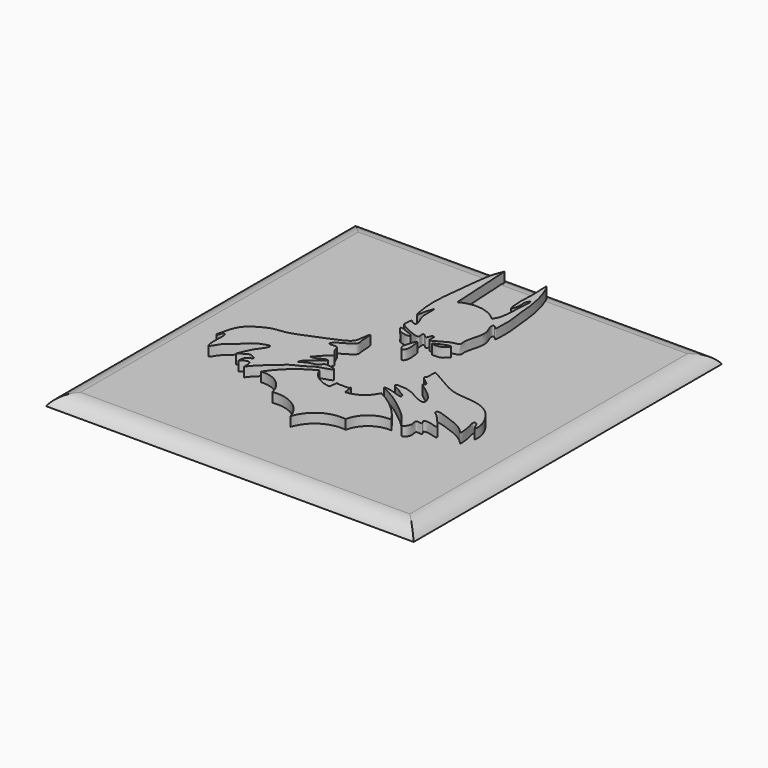
from build123d import *

# Parameters (mm, degrees)
F1_DEPTH    = 8.636
F0_W        = 157.6474606991
F0_H        = 165.2397401631
F2_DEPTH    = 4.572
F3_T1_DEPTH = 199.1265994465
F3_T3_DEPTH = 206.7188789105


# Not quite as in the source:
# - a fillet or chamfer that OpenCascade refuses, or shapes differently, is made with other operations: its cross-section is extruded or revolved along the edge and cut away or added


with BuildPart() as f1:
    # F0 (on Top) → F1 (new body)
    with BuildSketch(Plane.XY):
        with BuildLine():
            Line((-8.0563426018, 32.0382602513), (-9.5873847604, 59.3079030514))
            add(Edge.make_bspline(
                [(-9.5873847604, 59.3079030514), (-10.2069740501, 57.8510791752), (-11.6288952228, 54.5077536066), (-12.571011767, 45.9160526153), (-13.8278968188, 35.8790758133), (-14.8130812466, 24.4032074281), (-12.6930088149, 14.2813385529), (-12.4467480347, 19.5686321405), (-11.3588516792, 22.1258498776), (-10.9689455739, 23.9673491113), (-10.7703404995, 22.210055132), (-10.8849088261, 20.4345795664), (-10.8702437558, 16.7478927392), (-9.9164388242, 14.4470348521), (-8.9093176999, 12.4710831019), (-8.8130882414, 10.5507668204), (-10.0726759825, 11.0809174378), (-11.1105414789, 11.4684363429), (-11.5467394355, 12.4794641642), (-12.0326045569, 11.1352392958), (-12.0718164854, 9.0656207612), (-12.1678725214, 7.8042704483), (-1.7397194602, 2.850652627), (-2.7152347011, 5.6312047686), (-2.6333232506, 7.0837245523), (-1.5405587064, 6.595512113), (-0.3523573577, 5.1847846555), (0.0176657446, 6.1495776898), (0.3440615571, 6.8678292671), (0.6920890595, 7.6887216528), (1.7445455533, 7.8221392033), (1.6925707752, 6.6794200294), (1.5694466399, 5.9493515122), (1.7384837371, 5.3483126386), (1.7238072902, 4.2958486754), (4.2518249694, 5.5379971352), (7.5388645263, 7.6288405278), (9.5491214189, 8.2193902514), (12.1832042354, 8.6803960253), (11.2527745874, 11.5048248524), (12.9626901314, 16.4433777124), (13.6012979663, 21.5049566899), (11.6736068309, 24.314855315), (11.7201059386, 26.9225111344), (13.2570231691, 25.7198167097), (14.0571000334, 24.3610756973), (14.1651481676, 28.6480973338), (14.2838550528, 32.7466596802), (13.191654245, 38.6947421466), (13.0597426804, 43.5898107344), (11.6516605619, 52.5903286162), (7.7032874495, 61.6806237813), (8.3342558909, 55.6029864465), (8.3560371943, 48.142569085), (7.9148713681, 45.9656915319), (8.3982670386, 41.7710296595), (8.7042650126, 38.596342426), (10.3088253456, 43.154016532), (9.3465585879, 45.7452585782), (11.2795851261, 48.6649542065), (10.9361180212, 44.1687097023), (10.5666606894, 40.3809380114), (10.4802282511, 32.4778899259), (8.6848033832, 30.3255504932), (8.5917155195, 29.9147238101), (8.5641695186, 29.7931544483)],
                knots=[0, 0, 0, 0, 0.0215680204, 0.0494973451, 0.0803067556, 0.1149771587, 0.1397760921, 0.1556042663, 0.173574449, 0.1833185564, 0.1930074754, 0.2067732445, 0.2250113268, 0.2403192089, 0.2549776383, 0.2662207325, 0.2755793133, 0.2862530722, 0.2940626367, 0.3034624078, 0.3174077042, 0.3281447576, 0.3578417858, 0.368882565, 0.3793332655, 0.3883559951, 0.400307943, 0.4079673083, 0.4169542407, 0.425807678, 0.4339422803, 0.4431398948, 0.4516444118, 0.4593494611, 0.4669484468, 0.4812481254, 0.5008700638, 0.5152502277, 0.5289135867, 0.5433599989, 0.5656053014, 0.5871321546, 0.6049528358, 0.6172889038, 0.6286238669, 0.6374714134, 0.6542574113, 0.6752363731, 0.698287396, 0.7195672617, 0.7501912632, 0.7750519975, 0.7925526419, 0.8197608492, 0.8345022352, 0.8547565152, 0.8673256205, 0.8844942075, 0.9019948421, 0.9149074029, 0.9308938897, 0.9517413657, 0.9785266178, 0.9936457258, 1, 1, 1, 1], degree=3))
            ThreePointArc((8.5641695186, 29.7931544483), (0.6273246637, 33.6800694814), (-8.0563426018, 32.0382602513))
        make_face()
    extrude(amount=F1_DEPTH)


with BuildPart() as f1b:
    # F0 (on Top) → F1, piece 2 (new body)
    with BuildSketch(Plane.XY):
        with BuildLine():
            add(Edge.make_bspline(
                [(-11.3129224628, 5.8338870294), (-11.212077991, 6.0836919569), (-9.5446702313, 5.498751424), (-7.6526266007, 4.7544780652), (-4.8522655809, 3.7151044125), (-5.6744214857, 2.3720213293), (-8.5846141026, 3.1775841412), (-9.7788566178, 3.3609961858), (-11.4458218222, 5.5046779591), (-11.3129224628, 5.8338870294)],
                knots=[0, 0, 0, 0, 0.1234585709, 0.2884281256, 0.4484905967, 0.5401562643, 0.7088422597, 0.83729832, 1, 1, 1, 1], degree=3))
        make_face()
    extrude(amount=F1_DEPTH)


with BuildPart() as f1c:
    # F0 (on Top) → F1, piece 3 (new body)
    with BuildSketch(Plane.XY):
        with BuildLine():
            add(Edge.make_bspline(
                [(4.2034736834, 3.2082463149), (4.1171338962, 3.3867294322), (5.3945718393, 4.2279527832), (7.871360839, 5.2078627509), (9.5517951768, 5.8839128476), (10.8777071041, 5.6073678199), (9.2708457074, 4.4751151628), (8.2710626919, 3.2190418207), (6.3604336283, 3.0183269191), (4.3102453409, 2.9875260782), (4.2034736834, 3.2082463149)],
                knots=[0, 0, 0, 0, 0.1086692497, 0.274727001, 0.406939114, 0.4888761294, 0.6034499567, 0.727631672, 0.8656147266, 1, 1, 1, 1], degree=3))
        make_face()
    extrude(amount=F1_DEPTH)


with BuildPart() as f1d:
    # F0 (on Top) → F1, piece 4 (new body)
    with BuildSketch(Plane.XY):
        with BuildLine():
            add(Edge.make_bspline(
                [(-0.4922925145, 1.1984186713), (-0.7219822659, 1.2413124065), (-1.5725812282, -0.1617702452), (-1.8935343811, -2.3371597334), (-2.5761843842, -3.8672516478), (-2.3162609098, -5.1141898438), (-1.0121639923, -6.7835477453), (0.4038948302, -4.6520691166), (-0.0283463576, -1.1777215689), (-0.0962722826, 0.1357641207), (-0.3086551187, 1.1641250479), (-0.4922925145, 1.1984186713)],
                knots=[0, 0, 0, 0, 0.102513173, 0.2351976422, 0.3413296648, 0.4367849301, 0.5411400619, 0.6544107074, 0.8137842706, 0.918040522, 1, 1, 1, 1], degree=3))
        make_face()
    extrude(amount=F1_DEPTH)


with BuildPart() as f1e:
    # F0 (on Top) → F1, piece 5 (new body)
    with BuildSketch(Plane.XY):
        with BuildLine():
            add(Edge.make_bspline(
                [(-56.5317720175, -36.4757142961), (-56.3085275842, -35.3899332292), (-55.7960366931, -32.8885452847), (-54.0426175772, -26.7831440592), (-48.5321006344, -23.2926451301), (-44.5299851578, -21.2785733802), (-37.744733397, -21.0053075427), (-30.8060554473, -17.4194604059), (-18.5940164844, -13.2184714608), (-16.8743985097, -10.1721897893), (-16.9012842846, -7.8020298205), (-15.8976571712, -3.1934213643), (-15.8006185861, -7.4747740916), (-15.7020221735, -9.8808797844), (-15.036609521, -11.83844459), (-16.4503720124, -13.4391939901), (-20.0262562132, -15.3997435363), (-21.8881261976, -16.2977734279), (-23.3955349466, -18.4890981482), (-21.0565555139, -18.3918166801), (-19.0412600912, -18.140499788), (-18.8028673653, -19.8230302625), (-17.818011388, -21.6935992037), (-17.1193392555, -22.3536708663), (-15.7073878024, -24.0554988779), (-18.7233056749, -25.7252328416), (-20.3645373071, -28.354481793), (-22.8099407509, -29.9214724173), (-18.7229926684, -29.1680810509), (-17.5001874468, -27.941324871), (-14.3629528526, -27.486134602), (-18.6008603941, -30.3633212973), (-20.0842758034, -31.8567752366), (-21.9914900575, -32.9897828812), (-23.3175952088, -35.9553450316), (-19.9363871131, -32.9237966924), (-15.3834104243, -32.8316576362), (-15.2787570435, -30.6204718377), (-12.5601866802, -30.5905559397), (-8.5162795966, -31.8659123733), (-12.8665495258, -33.1359132687), (-16.3544489489, -34.1340040074), (-19.6077369159, -36.8480297152), (-23.9258639487, -38.2572226049), (-26.4016508932, -41.3086310679), (-29.889560769, -43.7575731288), (-33.2428135147, -47.1877803235), (-34.2014949385, -48.5179926444), (-34.5914438367, -49.0590669215)],
                knots=[0, 0, 0, 0, 0.0235054063, 0.0541714038, 0.0851440949, 0.111308795, 0.14222986, 0.1783242724, 0.2222777227, 0.2433825477, 0.2637111406, 0.2847053536, 0.3040919602, 0.3252304726, 0.3416503728, 0.3587446101, 0.3837110785, 0.4027046969, 0.4189237643, 0.434797145, 0.4516974638, 0.4663698249, 0.4842223365, 0.4970387457, 0.5124994639, 0.5331958128, 0.5567519831, 0.5718107872, 0.5922051865, 0.6111406286, 0.6263819983, 0.6496852012, 0.6694935076, 0.6882990399, 0.7047724597, 0.7262713232, 0.7524047523, 0.7671438816, 0.786982741, 0.807561723, 0.8283115693, 0.8533238079, 0.8784768485, 0.9045011258, 0.9285856605, 0.9544829455, 0.9815143267, 1, 1, 1, 1], degree=3))
            add(Edge.make_bspline(
                [(-34.5914438367, -49.0590669215), (-34.5617406662, -48.4645916409), (-34.5015091034, -47.2550371222), (-34.9231333712, -45.2879063315), (-36.6352958616, -45.0185438688), (-38.1275834761, -46.4156266116), (-39.0504091016, -47.1771096694), (-38.6387314573, -45.3877670548), (-38.4250127074, -43.1979119569), (-34.7845880016, -42.5577217331), (-37.7439039605, -40.9493748194), (-38.7560351456, -40.7890446139), (-40.8150603497, -42.1673004931), (-42.0745475807, -42.6956108287), (-42.8998646706, -43.8533010921), (-41.7082013729, -41.02927019), (-40.0292794785, -37.0379365322), (-37.3109398728, -33.9222730739), (-36.7235339468, -31.6524819302), (-38.8601120182, -31.9042472556), (-43.7324241455, -34.0352374035), (-46.2025642266, -37.594436589), (-49.9657372312, -40.1469617994), (-51.5753222919, -42.1336066798), (-53.3116998576, -45.5754431201), (-54.11435487, -42.6530847524), (-54.0795511785, -39.8375115199), (-53.9142722396, -36.9687224915), (-53.9337726693, -35.9541859846), (-54.3444092876, -34.0062490401), (-55.8776571006, -35.4763912856), (-55.773981613, -37.14106453), (-56.3128012293, -36.6679736125), (-56.5317720175, -36.4757142961)],
                knots=[0, 0, 0, 0, 0.0306089862, 0.0605779455, 0.0867220518, 0.119466043, 0.1379441871, 0.1633760962, 0.1971675416, 0.2306435809, 0.2632017867, 0.2874606202, 0.3216074169, 0.3496849568, 0.3678851507, 0.3995177636, 0.4492656593, 0.4956544404, 0.524008621, 0.55106341, 0.6027475455, 0.6504689503, 0.69697749, 0.735409776, 0.7717076052, 0.801572517, 0.8420773346, 0.8791897934, 0.9034034657, 0.9292672177, 0.9565885872, 0.981875991, 1, 1, 1, 1], degree=3))
        make_face()
    extrude(amount=F1_DEPTH)


with BuildPart() as f1f:
    # F0 (on Top) → F1, piece 6 (new body)
    with BuildSketch(Plane.XY):
        with BuildLine():
            add(Edge.make_bspline(
                [(11.3561199978, -31.5462760627), (11.2708232902, -31.8494182358), (17.1916397479, -34.2819237216), (22.8631387434, -38.8349813838), (29.8063616714, -44.1603330844), (33.1387713155, -50.1267706744), (34.5396741163, -48.8557368561), (35.4714882721, -47.213305576), (35.3042623997, -45.7627282077), (34.7935519176, -44.0431695576), (36.1375577984, -43.7628594372), (37.8716341978, -44.30387013), (37.4190158392, -43.159612785), (36.3824914624, -42.1406612695), (38.6318730978, -41.8072170173), (40.1553549966, -42.164726162), (44.0894732797, -43.5380661341), (41.4220220506, -40.4700964927), (39.3518408463, -38.0199885713), (37.3515430903, -35.8618404922), (35.9013185364, -35.1833512057), (36.3078265927, -33.5728204552), (39.4561495274, -34.6972965204), (44.3510012501, -36.2798979776), (50.0337333297, -38.8662677252), (52.1223899971, -42.0264216155), (51.989348781, -39.5219509981), (51.6582572588, -37.3685552937), (51.3032706529, -35.4106328984), (50.3378532171, -32.622045103), (51.7855547632, -32.2974748095), (52.6049629965, -33.6698853924), (53.9423638795, -37.048777693), (54.2409254928, -33.1267342607), (52.3854787877, -28.1337374698), (47.9530116507, -22.6083548802), (41.331769958, -20.5112354176), (35.05419088, -20.3961087662), (29.6940561643, -19.098259547), (24.1383301141, -15.832340626), (18.6607055154, -12.5331934369), (18.1259123911, -12.4097767417), (17.9909168325, -13.1479184713), (17.9535379241, -14.4114186042), (18.0676703856, -15.7004041283), (17.9260726891, -17.0669513695), (17.0850166317, -17.2757653009), (18.095102178, -18.4661333892), (19.9339732524, -19.6693085298), (21.1709176908, -20.8449222954), (20.8552869509, -21.7922559491), (19.5396603619, -21.5424004948), (21.1406348542, -22.760811599), (22.889906786, -23.8290796941), (24.9307608472, -25.6037416108), (25.3058857425, -25.7541587946), (27.2535142167, -27.7773825531), (27.5456715584, -28.0711397096), (28.3645450501, -29.6113323522), (28.9491463629, -31.2233535764), (27.7615827313, -31.9665108042), (25.6796017707, -31.1125851813), (23.7189459148, -30.3195990814), (20.868861509, -28.4078463352), (17.3597853751, -27.4504491891), (16.3649111705, -27.5741175461), (15.1791383287, -27.4827337621), (13.293302009, -27.2752369899), (13.2771080651, -28.8255516731), (16.4679377367, -29.5237431729), (17.6955882572, -31.2418041093), (19.902172027, -31.7891686271), (20.3497248586, -34.0562482813), (14.6119485045, -31.4979431235), (13.034312592, -31.4892860499), (11.3983533668, -31.3961798209), (11.3561199978, -31.5462760627)],
                knots=[0, 0, 0, 0, 0.0207712469, 0.0468010185, 0.0740281994, 0.0953806066, 0.1048831637, 0.1171105979, 0.1281810161, 0.1390164492, 0.1484333243, 0.1590379808, 0.1670070375, 0.1760829796, 0.1871520185, 0.2002205864, 0.2147618528, 0.2286747001, 0.2461395079, 0.2614180487, 0.2719585888, 0.2806602226, 0.2953583218, 0.3165908605, 0.3397066295, 0.3534940351, 0.3643098423, 0.3781409522, 0.3914439389, 0.405697964, 0.4137994303, 0.4254296768, 0.4393008252, 0.4524650877, 0.4739550989, 0.4974999134, 0.5208073503, 0.543208937, 0.5638870529, 0.5877483837, 0.6097735957, 0.6146449264, 0.6215906595, 0.6318524469, 0.6424545507, 0.6524798852, 0.6589274487, 0.6685474208, 0.6826281714, 0.6938838396, 0.701344386, 0.7089221438, 0.7188362561, 0.7331597297, 0.7472245684, 0.7538431679, 0.7683767168, 0.7749596765, 0.7865937658, 0.7978733074, 0.806796258, 0.8198580259, 0.8330984023, 0.8500047315, 0.8668764886, 0.8755687455, 0.8855328188, 0.8969508767, 0.9051905148, 0.9206295997, 0.9339190842, 0.9469970149, 0.9559339563, 0.9762144194, 0.9897154327, 1, 1, 1, 1], degree=3))
        make_face()
    extrude(amount=F1_DEPTH)


with BuildPart() as f1g:
    # F0 (on Top) → F1, piece 7 (new body)
    with BuildSketch(Plane.XY):
        with BuildLine():
            ThreePointArc((-3.3188456437, -42.3583795704), (-9.3072729106, -40.3191361107), (-13.2902822224, -35.4043205657))
            ThreePointArc((-13.2902822224, -35.4043205657), (-21.481283067, -40.8505875442), (-27.9277319787, -48.2800973036))
            ThreePointArc((-27.9277319787, -48.2800973036), (-20.0606479541, -50.5503244222), (-15.7425979851, -57.5072911956))
            ThreePointArc((-15.7425979851, -57.5072911956), (-6.0369640986, -59.5197584467), (0, -67.3813370444))
            ThreePointArc((0, -67.3813370444), (6.0369640986, -59.5197584467), (15.7425979851, -57.5072911956))
            ThreePointArc((15.7425979851, -57.5072911956), (20.0606479541, -50.5503244222), (27.9277319787, -48.2800973036))
            ThreePointArc((27.9277319787, -48.2800973036), (21.481283067, -40.8505875442), (13.2902822224, -35.4043205657))
            ThreePointArc((13.2902822224, -35.4043205657), (9.3072729106, -40.3191361107), (3.3188456437, -42.3583795704))
            Line((3.3188456437, -42.3583795704), (2.8344087768, -38.5856293142))
            Line((2.8344087768, -38.5856293142), (2.3823640459, -39.2272426674))
            Line((2.3823640459, -39.2272426674), (0, -39.2272426674))
            Line((0, -39.2272426674), (-2.3823640459, -39.2272426674))
            Line((-2.3823640459, -39.2272426674), (-2.8344087768, -38.5856293142))
            Line((-2.8344087768, -38.5856293142), (-3.3188456437, -42.3583795704))
        make_face()
    extrude(amount=F1_DEPTH)


with BuildPart() as f2:
    # F0 (on Top) → F2 (new body)
    with BuildSketch(Plane.XY):
        with Locations((0, -17.3164587468)):
            Rectangle(F0_W, F0_H)
        with BuildLine():
            add(Edge.make_bspline(
                [(-34.5914438367, -49.0590669215), (-34.5617406662, -48.4645916409), (-34.5015091034, -47.2550371222), (-34.9231333712, -45.2879063315), (-36.6352958616, -45.0185438688), (-38.1275834761, -46.4156266116), (-39.0504091016, -47.1771096694), (-38.6387314573, -45.3877670548), (-38.4250127074, -43.1979119569), (-34.7845880016, -42.5577217331), (-37.7439039605, -40.9493748194), (-38.7560351456, -40.7890446139), (-40.8150603497, -42.1673004931), (-42.0745475807, -42.6956108287), (-42.8998646706, -43.8533010921), (-41.7082013729, -41.02927019), (-40.0292794785, -37.0379365322), (-37.3109398728, -33.9222730739), (-36.7235339468, -31.6524819302), (-38.8601120182, -31.9042472556), (-43.7324241455, -34.0352374035), (-46.2025642266, -37.594436589), (-49.9657372312, -40.1469617994), (-51.5753222919, -42.1336066798), (-53.3116998576, -45.5754431201), (-54.11435487, -42.6530847524), (-54.0795511785, -39.8375115199), (-53.9142722396, -36.9687224915), (-53.9337726693, -35.9541859846), (-54.3444092876, -34.0062490401), (-55.8776571006, -35.4763912856), (-55.773981613, -37.14106453), (-56.3128012293, -36.6679736125), (-56.5317720175, -36.4757142961)],
                knots=[0, 0, 0, 0, 0.0306089862, 0.0605779455, 0.0867220518, 0.119466043, 0.1379441871, 0.1633760962, 0.1971675416, 0.2306435809, 0.2632017867, 0.2874606202, 0.3216074169, 0.3496849568, 0.3678851507, 0.3995177636, 0.4492656593, 0.4956544404, 0.524008621, 0.55106341, 0.6027475455, 0.6504689503, 0.69697749, 0.735409776, 0.7717076052, 0.801572517, 0.8420773346, 0.8791897934, 0.9034034657, 0.9292672177, 0.9565885872, 0.981875991, 1, 1, 1, 1], degree=3))
            add(Edge.make_bspline(
                [(-56.5317720175, -36.4757142961), (-56.3085275842, -35.3899332292), (-55.7960366931, -32.8885452847), (-54.0426175772, -26.7831440592), (-48.5321006344, -23.2926451301), (-44.5299851578, -21.2785733802), (-37.744733397, -21.0053075427), (-30.8060554473, -17.4194604059), (-18.5940164844, -13.2184714608), (-16.8743985097, -10.1721897893), (-16.9012842846, -7.8020298205), (-15.8976571712, -3.1934213643), (-15.8006185861, -7.4747740916), (-15.7020221735, -9.8808797844), (-15.036609521, -11.83844459), (-16.4503720124, -13.4391939901), (-20.0262562132, -15.3997435363), (-21.8881261976, -16.2977734279), (-23.3955349466, -18.4890981482), (-21.0565555139, -18.3918166801), (-19.0412600912, -18.140499788), (-18.8028673653, -19.8230302625), (-17.818011388, -21.6935992037), (-17.1193392555, -22.3536708663), (-15.7073878024, -24.0554988779), (-18.7233056749, -25.7252328416), (-20.3645373071, -28.354481793), (-22.8099407509, -29.9214724173), (-18.7229926684, -29.1680810509), (-17.5001874468, -27.941324871), (-14.3629528526, -27.486134602), (-18.6008603941, -30.3633212973), (-20.0842758034, -31.8567752366), (-21.9914900575, -32.9897828812), (-23.3175952088, -35.9553450316), (-19.9363871131, -32.9237966924), (-15.3834104243, -32.8316576362), (-15.2787570435, -30.6204718377), (-12.5601866802, -30.5905559397), (-8.5162795966, -31.8659123733), (-12.8665495258, -33.1359132687), (-16.3544489489, -34.1340040074), (-19.6077369159, -36.8480297152), (-23.9258639487, -38.2572226049), (-26.4016508932, -41.3086310679), (-29.889560769, -43.7575731288), (-33.2428135147, -47.1877803235), (-34.2014949385, -48.5179926444), (-34.5914438367, -49.0590669215)],
                knots=[0, 0, 0, 0, 0.0235054063, 0.0541714038, 0.0851440949, 0.111308795, 0.14222986, 0.1783242724, 0.2222777227, 0.2433825477, 0.2637111406, 0.2847053536, 0.3040919602, 0.3252304726, 0.3416503728, 0.3587446101, 0.3837110785, 0.4027046969, 0.4189237643, 0.434797145, 0.4516974638, 0.4663698249, 0.4842223365, 0.4970387457, 0.5124994639, 0.5331958128, 0.5567519831, 0.5718107872, 0.5922051865, 0.6111406286, 0.6263819983, 0.6496852012, 0.6694935076, 0.6882990399, 0.7047724597, 0.7262713232, 0.7524047523, 0.7671438816, 0.786982741, 0.807561723, 0.8283115693, 0.8533238079, 0.8784768485, 0.9045011258, 0.9285856605, 0.9544829455, 0.9815143267, 1, 1, 1, 1], degree=3))
        make_face(mode=Mode.SUBTRACT)
        with BuildLine():
            ThreePointArc((-27.9277319787, -48.2800973036), (-21.481283067, -40.8505875442), (-13.2902822224, -35.4043205657))
            ThreePointArc((-13.2902822224, -35.4043205657), (-9.3072729106, -40.3191361107), (-3.3188456437, -42.3583795704))
            Line((-3.3188456437, -42.3583795704), (-2.8344087768, -38.5856293142))
            Line((-2.8344087768, -38.5856293142), (-2.3823640459, -39.2272426674))
            Line((-2.3823640459, -39.2272426674), (0, -39.2272426674))
            Line((0, -39.2272426674), (2.3823640459, -39.2272426674))
            Line((2.3823640459, -39.2272426674), (2.8344087768, -38.5856293142))
            Line((2.8344087768, -38.5856293142), (3.3188456437, -42.3583795704))
            ThreePointArc((3.3188456437, -42.3583795704), (9.3072729106, -40.3191361107), (13.2902822224, -35.4043205657))
            ThreePointArc((13.2902822224, -35.4043205657), (21.481283067, -40.8505875442), (27.9277319787, -48.2800973036))
            ThreePointArc((27.9277319787, -48.2800973036), (20.0606479541, -50.5503244222), (15.7425979851, -57.5072911956))
            ThreePointArc((15.7425979851, -57.5072911956), (6.0369640986, -59.5197584467), (0, -67.3813370444))
            ThreePointArc((0, -67.3813370444), (-6.0369640986, -59.5197584467), (-15.7425979851, -57.5072911956))
            ThreePointArc((-15.7425979851, -57.5072911956), (-20.0606479541, -50.5503244222), (-27.9277319787, -48.2800973036))
        make_face(mode=Mode.SUBTRACT)
        with BuildLine():
            add(Edge.make_bspline(
                [(11.3561199978, -31.5462760627), (11.2708232902, -31.8494182358), (17.1916397479, -34.2819237216), (22.8631387434, -38.8349813838), (29.8063616714, -44.1603330844), (33.1387713155, -50.1267706744), (34.5396741163, -48.8557368561), (35.4714882721, -47.213305576), (35.3042623997, -45.7627282077), (34.7935519176, -44.0431695576), (36.1375577984, -43.7628594372), (37.8716341978, -44.30387013), (37.4190158392, -43.159612785), (36.3824914624, -42.1406612695), (38.6318730978, -41.8072170173), (40.1553549966, -42.164726162), (44.0894732797, -43.5380661341), (41.4220220506, -40.4700964927), (39.3518408463, -38.0199885713), (37.3515430903, -35.8618404922), (35.9013185364, -35.1833512057), (36.3078265927, -33.5728204552), (39.4561495274, -34.6972965204), (44.3510012501, -36.2798979776), (50.0337333297, -38.8662677252), (52.1223899971, -42.0264216155), (51.989348781, -39.5219509981), (51.6582572588, -37.3685552937), (51.3032706529, -35.4106328984), (50.3378532171, -32.622045103), (51.7855547632, -32.2974748095), (52.6049629965, -33.6698853924), (53.9423638795, -37.048777693), (54.2409254928, -33.1267342607), (52.3854787877, -28.1337374698), (47.9530116507, -22.6083548802), (41.331769958, -20.5112354176), (35.05419088, -20.3961087662), (29.6940561643, -19.098259547), (24.1383301141, -15.832340626), (18.6607055154, -12.5331934369), (18.1259123911, -12.4097767417), (17.9909168325, -13.1479184713), (17.9535379241, -14.4114186042), (18.0676703856, -15.7004041283), (17.9260726891, -17.0669513695), (17.0850166317, -17.2757653009), (18.095102178, -18.4661333892), (19.9339732524, -19.6693085298), (21.1709176908, -20.8449222954), (20.8552869509, -21.7922559491), (19.5396603619, -21.5424004948), (21.1406348542, -22.760811599), (22.889906786, -23.8290796941), (24.9307608472, -25.6037416108), (25.3058857425, -25.7541587946), (27.2535142167, -27.7773825531), (27.5456715584, -28.0711397096), (28.3645450501, -29.6113323522), (28.9491463629, -31.2233535764), (27.7615827313, -31.9665108042), (25.6796017707, -31.1125851813), (23.7189459148, -30.3195990814), (20.868861509, -28.4078463352), (17.3597853751, -27.4504491891), (16.3649111705, -27.5741175461), (15.1791383287, -27.4827337621), (13.293302009, -27.2752369899), (13.2771080651, -28.8255516731), (16.4679377367, -29.5237431729), (17.6955882572, -31.2418041093), (19.902172027, -31.7891686271), (20.3497248586, -34.0562482813), (14.6119485045, -31.4979431235), (13.034312592, -31.4892860499), (11.3983533668, -31.3961798209), (11.3561199978, -31.5462760627)],
                knots=[0, 0, 0, 0, 0.0207712469, 0.0468010185, 0.0740281994, 0.0953806066, 0.1048831637, 0.1171105979, 0.1281810161, 0.1390164492, 0.1484333243, 0.1590379808, 0.1670070375, 0.1760829796, 0.1871520185, 0.2002205864, 0.2147618528, 0.2286747001, 0.2461395079, 0.2614180487, 0.2719585888, 0.2806602226, 0.2953583218, 0.3165908605, 0.3397066295, 0.3534940351, 0.3643098423, 0.3781409522, 0.3914439389, 0.405697964, 0.4137994303, 0.4254296768, 0.4393008252, 0.4524650877, 0.4739550989, 0.4974999134, 0.5208073503, 0.543208937, 0.5638870529, 0.5877483837, 0.6097735957, 0.6146449264, 0.6215906595, 0.6318524469, 0.6424545507, 0.6524798852, 0.6589274487, 0.6685474208, 0.6826281714, 0.6938838396, 0.701344386, 0.7089221438, 0.7188362561, 0.7331597297, 0.7472245684, 0.7538431679, 0.7683767168, 0.7749596765, 0.7865937658, 0.7978733074, 0.806796258, 0.8198580259, 0.8330984023, 0.8500047315, 0.8668764886, 0.8755687455, 0.8855328188, 0.8969508767, 0.9051905148, 0.9206295997, 0.9339190842, 0.9469970149, 0.9559339563, 0.9762144194, 0.9897154327, 1, 1, 1, 1], degree=3))
        make_face(mode=Mode.SUBTRACT)
        with BuildLine():
            add(Edge.make_bspline(
                [(-0.4922925145, 1.1984186713), (-0.7219822659, 1.2413124065), (-1.5725812282, -0.1617702452), (-1.8935343811, -2.3371597334), (-2.5761843842, -3.8672516478), (-2.3162609098, -5.1141898438), (-1.0121639923, -6.7835477453), (0.4038948302, -4.6520691166), (-0.0283463576, -1.1777215689), (-0.0962722826, 0.1357641207), (-0.3086551187, 1.1641250479), (-0.4922925145, 1.1984186713)],
                knots=[0, 0, 0, 0, 0.102513173, 0.2351976422, 0.3413296648, 0.4367849301, 0.5411400619, 0.6544107074, 0.8137842706, 0.918040522, 1, 1, 1, 1], degree=3))
        make_face(mode=Mode.SUBTRACT)
        with BuildLine():
            add(Edge.make_bspline(
                [(-11.3129224628, 5.8338870294), (-11.212077991, 6.0836919569), (-9.5446702313, 5.498751424), (-7.6526266007, 4.7544780652), (-4.8522655809, 3.7151044125), (-5.6744214857, 2.3720213293), (-8.5846141026, 3.1775841412), (-9.7788566178, 3.3609961858), (-11.4458218222, 5.5046779591), (-11.3129224628, 5.8338870294)],
                knots=[0, 0, 0, 0, 0.1234585709, 0.2884281256, 0.4484905967, 0.5401562643, 0.7088422597, 0.83729832, 1, 1, 1, 1], degree=3))
        make_face(mode=Mode.SUBTRACT)
        with BuildLine():
            add(Edge.make_bspline(
                [(-9.5873847604, 59.3079030514), (-10.2069740501, 57.8510791752), (-11.6288952228, 54.5077536066), (-12.571011767, 45.9160526153), (-13.8278968188, 35.8790758133), (-14.8130812466, 24.4032074281), (-12.6930088149, 14.2813385529), (-12.4467480347, 19.5686321405), (-11.3588516792, 22.1258498776), (-10.9689455739, 23.9673491113), (-10.7703404995, 22.210055132), (-10.8849088261, 20.4345795664), (-10.8702437558, 16.7478927392), (-9.9164388242, 14.4470348521), (-8.9093176999, 12.4710831019), (-8.8130882414, 10.5507668204), (-10.0726759825, 11.0809174378), (-11.1105414789, 11.4684363429), (-11.5467394355, 12.4794641642), (-12.0326045569, 11.1352392958), (-12.0718164854, 9.0656207612), (-12.1678725214, 7.8042704483), (-1.7397194602, 2.850652627), (-2.7152347011, 5.6312047686), (-2.6333232506, 7.0837245523), (-1.5405587064, 6.595512113), (-0.3523573577, 5.1847846555), (0.0176657446, 6.1495776898), (0.3440615571, 6.8678292671), (0.6920890595, 7.6887216528), (1.7445455533, 7.8221392033), (1.6925707752, 6.6794200294), (1.5694466399, 5.9493515122), (1.7384837371, 5.3483126386), (1.7238072902, 4.2958486754), (4.2518249694, 5.5379971352), (7.5388645263, 7.6288405278), (9.5491214189, 8.2193902514), (12.1832042354, 8.6803960253), (11.2527745874, 11.5048248524), (12.9626901314, 16.4433777124), (13.6012979663, 21.5049566899), (11.6736068309, 24.314855315), (11.7201059386, 26.9225111344), (13.2570231691, 25.7198167097), (14.0571000334, 24.3610756973), (14.1651481676, 28.6480973338), (14.2838550528, 32.7466596802), (13.191654245, 38.6947421466), (13.0597426804, 43.5898107344), (11.6516605619, 52.5903286162), (7.7032874495, 61.6806237813), (8.3342558909, 55.6029864465), (8.3560371943, 48.142569085), (7.9148713681, 45.9656915319), (8.3982670386, 41.7710296595), (8.7042650126, 38.596342426), (10.3088253456, 43.154016532), (9.3465585879, 45.7452585782), (11.2795851261, 48.6649542065), (10.9361180212, 44.1687097023), (10.5666606894, 40.3809380114), (10.4802282511, 32.4778899259), (8.6848033832, 30.3255504932), (8.5917155195, 29.9147238101), (8.5641695186, 29.7931544483)],
                knots=[0, 0, 0, 0, 0.0215680204, 0.0494973451, 0.0803067556, 0.1149771587, 0.1397760921, 0.1556042663, 0.173574449, 0.1833185564, 0.1930074754, 0.2067732445, 0.2250113268, 0.2403192089, 0.2549776383, 0.2662207325, 0.2755793133, 0.2862530722, 0.2940626367, 0.3034624078, 0.3174077042, 0.3281447576, 0.3578417858, 0.368882565, 0.3793332655, 0.3883559951, 0.400307943, 0.4079673083, 0.4169542407, 0.425807678, 0.4339422803, 0.4431398948, 0.4516444118, 0.4593494611, 0.4669484468, 0.4812481254, 0.5008700638, 0.5152502277, 0.5289135867, 0.5433599989, 0.5656053014, 0.5871321546, 0.6049528358, 0.6172889038, 0.6286238669, 0.6374714134, 0.6542574113, 0.6752363731, 0.698287396, 0.7195672617, 0.7501912632, 0.7750519975, 0.7925526419, 0.8197608492, 0.8345022352, 0.8547565152, 0.8673256205, 0.8844942075, 0.9019948421, 0.9149074029, 0.9308938897, 0.9517413657, 0.9785266178, 0.9936457258, 1, 1, 1, 1], degree=3))
            Line((-9.5873847604, 59.3079030514), (-8.0563426018, 32.0382602513))
            ThreePointArc((-8.0563426018, 32.0382602513), (0.6273246637, 33.6800694814), (8.5641695186, 29.7931544483))
        make_face(mode=Mode.SUBTRACT)
        with BuildLine():
            add(Edge.make_bspline(
                [(4.2034736834, 3.2082463149), (4.1171338962, 3.3867294322), (5.3945718393, 4.2279527832), (7.871360839, 5.2078627509), (9.5517951768, 5.8839128476), (10.8777071041, 5.6073678199), (9.2708457074, 4.4751151628), (8.2710626919, 3.2190418207), (6.3604336283, 3.0183269191), (4.3102453409, 2.9875260782), (4.2034736834, 3.2082463149)],
                knots=[0, 0, 0, 0, 0.1086692497, 0.274727001, 0.406939114, 0.4888761294, 0.6034499567, 0.727631672, 0.8656147266, 1, 1, 1, 1], degree=3))
        make_face(mode=Mode.SUBTRACT)
    extrude(amount=F2_DEPTH)

    # F3: fillet of radius 9.8113639175 on 4 edges, made by hand

    # F3_s2 → F3_t1 (cut)
    with BuildSketch(Plane.YZ.offset(-99.5632997232)):
        with BuildLine():
            ThreePointArc((-99.9366670081, 0.0002136222), (-96.3768302905, 3.3536710924), (-91.6405010885, 4.5724))
            Line((-91.6405010885, 4.5724), (-91.6405010885, 5.5536729603))
            ThreePointArc((-91.6405010885, 5.5536729603), (-95.7884149584, 5.5532729603), (-99.9363288283, 5.5532729603))
            Line((-99.9363288283, 5.5532729603), (-100.9176017886, 4.572))
            ThreePointArc((-100.9176017886, 4.572), (-100.9176017886, 2.2861068111), (-100.7662836, 0.5242679448))
            Line((-100.7662836, 0.5242679448), (-99.9366670081, 0.0002136222))
        make_face()
        with BuildLine():
            ThreePointArc((57.0075835949, 4.5724), (61.7439127969, 3.3536710924), (65.3037495145, 0.0002136222))
            Line((65.3037495145, 0.0002136222), (66.1333661065, 0.5242679448))
            ThreePointArc((66.1333661065, 0.5242679448), (66.284684295, 2.2861068111), (66.284684295, 4.572))
            Line((66.284684295, 4.572), (65.3034113348, 5.5532729603))
            ThreePointArc((65.3034113348, 5.5532729603), (61.1554974648, 5.5532729603), (57.0075835949, 5.5536729603))
            Line((57.0075835949, 5.5536729603), (57.0075835949, 4.5724))
        make_face()
    extrude(amount=F3_T1_DEPTH, mode=Mode.SUBTRACT)

    # F3_s4 → F3_t3 (cut)
    with BuildSketch(Plane.XZ.offset(-86.0429807085)):
        with BuildLine():
            ThreePointArc((70.5279026097, 4.5724), (75.2642318117, 3.3536710924), (78.8240685293, 0.0002136222))
            Line((78.8240685293, 0.0002136222), (79.6536851212, 0.5242679448))
            ThreePointArc((79.6536851212, 0.5242679448), (79.8050033098, 2.2861068111), (79.8050033098, 4.572))
            Line((79.8050033098, 4.572), (78.8237303495, 5.5532729603))
            ThreePointArc((78.8237303495, 5.5532729603), (74.6758164796, 5.5532729603), (70.5279026097, 5.5536729603))
            Line((70.5279026097, 5.5536729603), (70.5279026097, 4.5724))
        make_face()
        with BuildLine():
            ThreePointArc((-70.5279026097, 4.5724), (-75.2642318117, 3.3536710924), (-78.8240685293, 0.0002136222))
            Line((-78.8240685293, 0.0002136222), (-79.6536851212, 0.5242679448))
            ThreePointArc((-79.6536851212, 0.5242679448), (-79.8050033098, 2.2861068111), (-79.8050033098, 4.572))
            Line((-79.8050033098, 4.572), (-78.8237303495, 5.5532729603))
            ThreePointArc((-78.8237303495, 5.5532729603), (-74.6758164796, 5.5532729603), (-70.5279026097, 5.5536729603))
            Line((-70.5279026097, 5.5536729603), (-70.5279026097, 4.5724))
        make_face()
    extrude(amount=F3_T3_DEPTH, mode=Mode.SUBTRACT)


solid = Compound([f1.part, f1b.part, f1c.part, f1d.part, f1e.part, f1f.part, f1g.part, f2.part])
